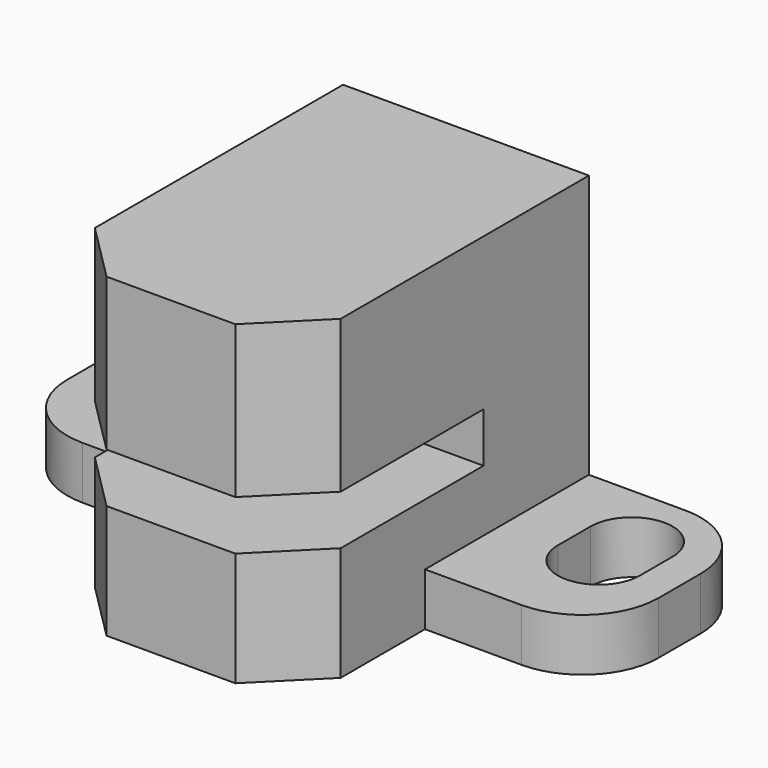
from build123d import *

# Parameters (mm, degrees)
F0_W     = 5.9
F0_H     = 7
F0_W_2   = 8.4
F1_DEPTH = 1.8
F0_H_2   = 5.6
F2_DEPTH = 10.8
F3_SIZE  = 2
F4_R     = 1
F5_DEPTH = 0.8
F7_DEPTH = 2.601
F8_W     = 2
F8_H     = 1.7
F8_W_2   = 6.1
F9_DEPTH = 14.301
F10_R    = 2.6


# Not quite as in the source:
# - a pattern or mirror of a feature is missing from the dataset's text; its kind, count and spacing are read off the source's solid


with BuildPart() as f1:
    # F0 (on Top) → F1 (new body)
    with BuildSketch(Plane.XY):
        with Locations((-7.15, -3.5)):
            Rectangle(F0_W, F0_H)
        with Locations((0, -3.5)):
            Rectangle(F0_W_2, F0_H)
        with Locations((7.15, -3.5)):
            Rectangle(F0_W, F0_H)
    extrude(amount=F1_DEPTH)

    # F0 (on Top) → F2 (join)
    with BuildSketch(Plane.XY):
        with Locations((0, -9.8)):
            Rectangle(F0_W_2, F0_H_2)
        with Locations((0, -3.5)):
            Rectangle(F0_W_2, F0_H)
    extrude(amount=F2_DEPTH)

    # F3
    f3_edges = [f1.edges().sort_by_distance(p)[0] for p in [
        (-4.2, -12.6, 5.4),
        (4.2, -12.6, 5.4),
    ]]
    chamfer(f3_edges, length=F3_SIZE)

    # F4 (on face) → F5 (join)
    with BuildSketch(Plane(origin=(0, 0, 0), x_dir=(1, 0, 0), z_dir=(0, 0, -1))):
        with Locations((0, 2.3)):
            Circle(F4_R)
        with Locations((0, 8.7)):
            Circle(F4_R)
    extrude(amount=F5_DEPTH)

    # F6 (on face) → F7 (cut, through all)
    with BuildSketch(Plane.XY.offset(1.8)):
        with BuildLine():
            Line((8.9, -3.7), (8.9, -2.3))
            ThreePointArc((8.9, -2.3), (7.5, -0.9), (6.1, -2.3))
            Line((6.1, -2.3), (6.1, -3.7))
            ThreePointArc((6.1, -3.7), (7.5, -5.1), (8.9, -3.7))
        make_face()
    f7 = extrude(amount=-F7_DEPTH, mode=Mode.SUBTRACT)

    # F7_copies: F7 across plane
    add(f7.mirror(Plane(origin=(0, 0, 0), x_dir=(0, 0, -1), z_dir=(-1, 0, 0))), mode=Mode.SUBTRACT)

    # F8 (on face) → F9 (cut, through all)
    with BuildSketch(Plane(origin=(-4.2, 0, 0), x_dir=(0, -1, 0), z_dir=(-1, 0, 0))):
        with Locations((11.6, 4.75)):
            Rectangle(F8_W, F8_H)
        with Locations((7.55, 4.75)):
            Rectangle(F8_W_2, F8_H)
    extrude(amount=-F9_DEPTH, mode=Mode.SUBTRACT)

    # F10
    f10_edges = [f1.edges().sort_by_distance(p)[0] for p in [
        (-10.1, -7, 0.9),
        (-10.1, 0, 0.9),
        (10.1, -7, 0.9),
        (10.1, 0, 0.9),
    ]]
    fillet(f10_edges, radius=F10_R)


solid = f1.part
